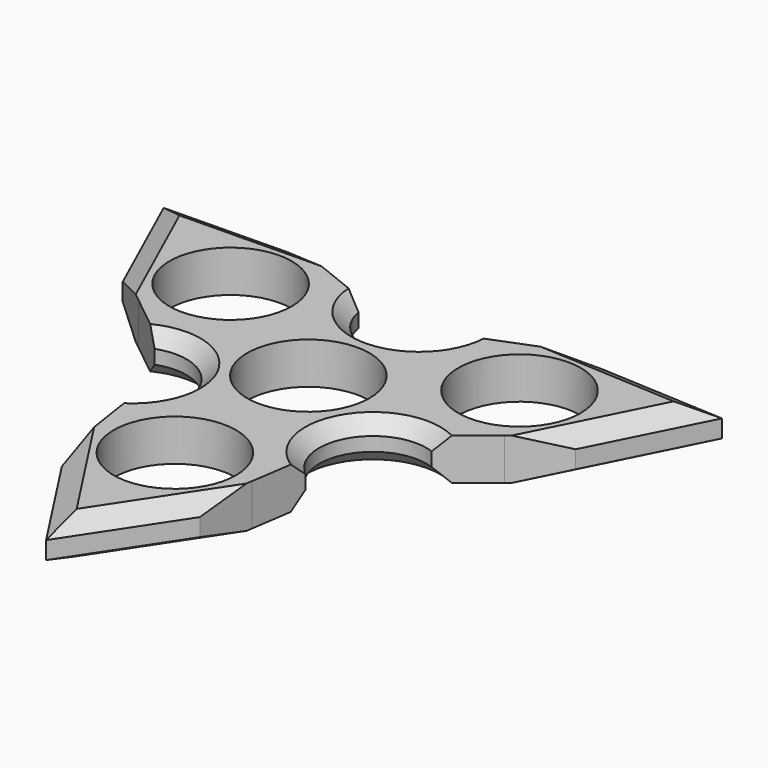
from build123d import *

# Parameters (mm, degrees)
F0_R       = 11.176
F1_DEPTH   = 7.62
F2_SIZE2   = 2.1997045256
F2_SIZE    = 3.81
F2_2_SIZE2 = 2.1997045256
F2_2_SIZE  = 3.81
F3_SIZE2   = 2.1997045256
F3_SIZE    = 3.81
F4_SIZE    = 2.54


# Not quite as in the source:
# - a feature names something its author has since deleted; it is built from what else it names


with BuildPart() as f1:
    # F0 (on Top) → F1 (new body)
    with BuildSketch(Plane.XY):
        with BuildLine():
            ThreePointArc((9.7057271537, 23.5283748909), (-0.0208649872, 15.4470615517), (-9.6943160077, 23.5919105566))
            Line((-9.6943160077, 23.5919105566), (-19.3886320155, 27.4654462223))
            Line((-19.3886320155, 27.4654462223), (-28.8233609262, 31.2352592656))
            Line((-28.8233609262, 31.2352592656), (-51.1347862104, 30.8821881406))
            Line((-51.1347862104, 30.8821881406), (-41.4352900784, 9.4122263494))
            Line((-41.4352900784, 9.4122263494), (-33.4914395336, 3.0781251091))
            Line((-33.4914395336, 3.0781251091), (-25.3390191684, -3.4222811682))
            ThreePointArc((-25.3390191684, -3.4222811682), (-13.4326493579, -7.7553437227), (-15.6332920147, -20.2330937227))
            Line((-15.6332920147, -20.2330937227), (-14.0799852263, -30.5435))
            Line((-14.0799852263, -30.5435), (-12.5664179144, -40.5901269958))
            Line((-12.5664179144, -40.5901269958), (-0.1099852263, -59.7535))
            Line((-0.1099852263, -59.7535), (12.5802445818, -40.4983495315))
            Line((12.5802445818, -40.4983495315), (14.0938118937, -30.4517225357))
            Line((14.0938118937, -30.4517225357), (15.6402053484, -20.1872049906))
            ThreePointArc((15.6402053484, -20.1872049906), (13.4326493579, -7.7553437227), (25.3027350274, -3.4512126568))
            Line((25.3027350274, -3.4512126568), (33.4188712518, 3.0202621318))
            Line((33.4188712518, 3.0202621318), (41.3627217965, 9.3543633721))
            Line((41.3627217965, 9.3543633721), (51.6930563519, 29.845))
            Line((51.6930563519, 29.845), (28.868872164, 31.0509006464))
            Line((28.868872164, 31.0509006464), (19.4114543073, 27.3383748909))
            Line((19.4114543073, 27.3383748909), (9.7057271537, 23.5283748909))
        make_face()
        with Locations((0, -30.48)):
            Circle(F0_R, mode=Mode.SUBTRACT)
        Circle(F0_R, mode=Mode.SUBTRACT)
        with Locations((-26.3964543073, 15.24)):
            Circle(F0_R, mode=Mode.SUBTRACT)
        with Locations((26.3964543073, 15.24)):
            Circle(F0_R, mode=Mode.SUBTRACT)
    extrude(amount=F1_DEPTH)

    # F2
    f2_edges = [f1.edges().sort_by_distance(p)[0] for p in [
        (-46.285038, 20.147207, 7.62),
        (-39.979074, 31.058724, 7.62),
        (40.280964, 30.44795, 7.62),
        (46.527889, 19.599682, 7.62),
        (6.23513, -50.125925, 7.62),
        (-6.338202, -50.171813, 7.62),
    ]]
    f2_side = f1.faces().sort_by_distance((19.789019, 26.011541, 7.62))[0]
    chamfer(f2_edges, length=F2_SIZE, length2=F2_SIZE2, reference=f2_side)

    # F2#2
    f2_2_edges = [f1.edges().sort_by_distance(p)[0] for p in [
        (-46.285038, 20.147207, 0),
        (46.527889, 19.599682, 0),
        (-39.979074, 31.058724, 0),
    ]]
    f2_2_side = f1.faces().sort_by_distance((19.789019, 26.011541, 0))[0]
    chamfer(f2_2_edges, length=F2_2_SIZE, length2=F2_2_SIZE2, reference=f2_2_side)

    # F3
    f3_edges = [f1.edges().sort_by_distance(p)[0] for p in [
        (-6.338202, -50.171813, 0),
        (6.23513, -50.125925, 0),
        (38.202915, 30.557743, 0),
    ]]
    f3_side = f1.faces().sort_by_distance((-15.154017, 24.375179, 0))[0]
    chamfer(f3_edges, length=F3_SIZE, length2=F3_SIZE2, reference=f3_side)

    # F4
    f4_edges = [f1.edges().sort_by_distance(p)[0] for p in [
        (-0.020865, 15.447062, 7.62),
        (13.432649, -7.755344, 7.62),
        (-13.432649, -7.755344, 7.62),
        (-13.432649, -7.755344, 0),
        (-0.020865, 15.447062, 0),
        (13.432649, -7.755344, 0),
    ]]
    chamfer(f4_edges, length=F4_SIZE)


solid = f1.part
